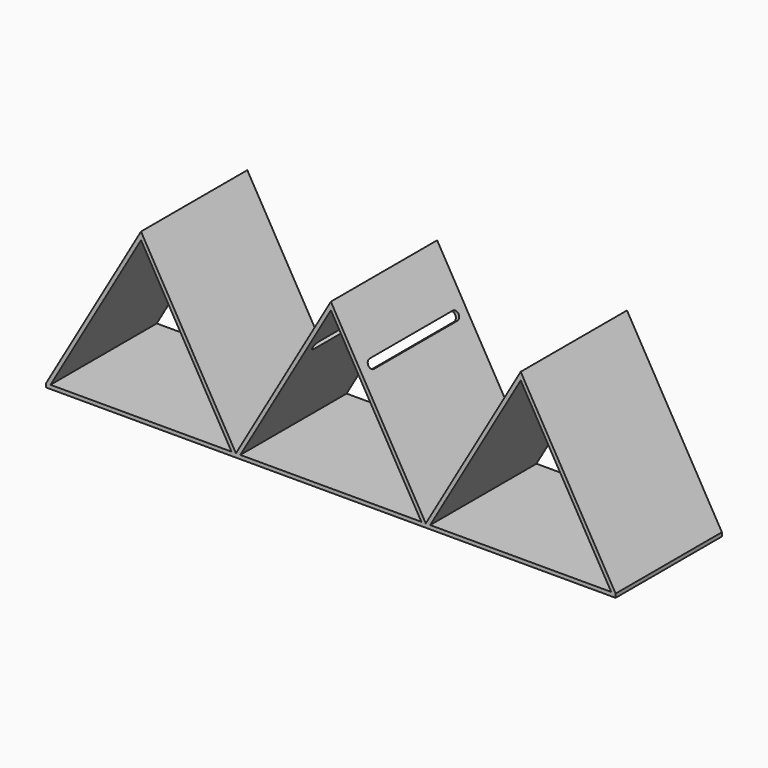
from build123d import *

# Parameters (mm, degrees)
F1_DEPTH = 105
F4_DEPTH = 3
F5_DEPTH = 3.2


with BuildPart() as f1:
    # F0 (on Front) → F1 (new body)
    with BuildSketch(Plane.XZ):
        Polygon((31.5868725905, 38.7087155582), (-43.4131274095, -91.1950950095), (-39.9490257943, -91.1950950095), (31.5868725905, 32.7087155582), (103.1227709754, -91.1950950095), (106.5868725905, -91.1950950095), align=None)
        Polygon((181.5868725905, 38.7087155582), (106.5868725905, -91.1950950095), (110.0509742057, -91.1950950095), (181.5868725905, 32.7087155582), (253.1227709754, -91.1950950095), (256.5868725905, -91.1950950095), align=None)
        Polygon((403.1227709754, -91.1950950095), (406.5868725905, -91.1950950095), (331.5868725905, 38.7087155582), (256.5868725905, -91.1950950095), (260.0509742057, -91.1950950095), (331.5868725905, 32.7087155582), align=None)
        Polygon((-39.9490257943, -91.1950950095), (-43.4131274095, -91.1950950095), (-43.3987992861, -94.1795955126), (406.5868725905, -94.1795955126), (406.5868725905, -91.1950950095), (403.1227709754, -91.1950950095), (260.0509742057, -91.1950950095), (256.5868725905, -91.1950950095), (253.1227709754, -91.1950950095), (110.0509742057, -91.1950950095), (106.5868725905, -91.1950950095), (103.1227709754, -91.1950950095), align=None)
    extrude(amount=F1_DEPTH)

    # F2 (on face) → F4 (cut)
    with BuildSketch(Plane(origin=(152.9515199535, 0, 88.3066012181), x_dir=(0, 1, 0), z_dir=(0.8660254038, 0, 0.5))):
        with BuildLine():
            Line((-11.2848039716, -100.270705274), (-93.8924178481, -100.270705274))
            ThreePointArc((-93.8924178481, -100.270705274), (-97, -103.770705274), (-93.8924178481, -107.270705274))
            Line((-93.8924178481, -107.270705274), (-10.656950064, -107.270705274))
            ThreePointArc((-10.656950064, -107.270705274), (-8.0142508316, -103.5055153734), (-11.2848039716, -100.270705274))
        make_face()
    extrude(amount=-F4_DEPTH, mode=Mode.SUBTRACT)

    # F3 (on face) → F5 (cut)
    with BuildSketch(Plane(origin=(119.4287889323, 0, -68.952243439), x_dir=(0, -1, 0), z_dir=(-0.8660254038, 0, 0.5))):
        with BuildLine():
            Line((93.957901001, 81.3161673165), (10.8784036711, 81.3161673165))
            ThreePointArc((10.8784036711, 81.3161673165), (8.0006789358, 77.7585614935), (11.0152736306, 74.3161673165))
            Line((11.0152736306, 74.3161673165), (94.2316353321, 74.3161673165))
            ThreePointArc((94.2316353321, 74.3161673165), (96.9972779307, 77.9296696835), (93.957901001, 81.3161673165))
        make_face()
    extrude(amount=-F5_DEPTH, mode=Mode.SUBTRACT)


solid = f1.part
